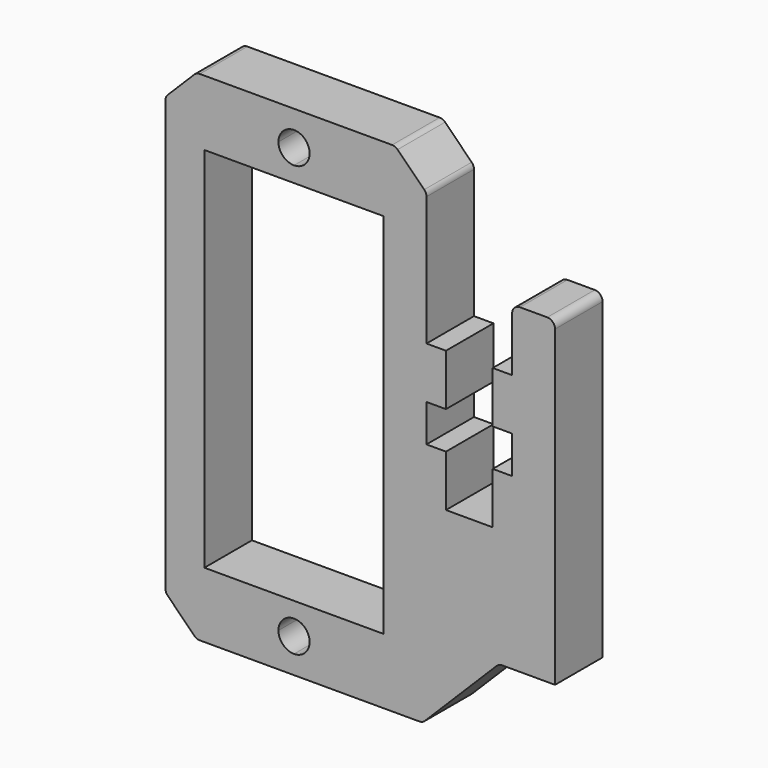
from build123d import *

# Parameters (mm, degrees)
F1_DEPTH = 3.81


# Not quite as in the source:
# - ends of sketch curves that miss each other by under 0.0002 mm in the source are joined


with BuildPart() as f1:
    # F0 (on Front) → F1 (new body)
    with BuildSketch(Plane.XZ):
        with BuildLine():
            Line((-10.292893, -16), (-4.25, -16))
            Line((-4.25, -16), (-4.25, -14.8))
            ThreePointArc((-4.25, -14.8), (-4.9571067812, -14.5071067812), (-5.25, -13.8))
            ThreePointArc((-5.25, -13.8), (-4.9571067812, -13.0928932188), (-4.25, -12.8))
            Line((-4.25, -12.8), (-4.25, -11.8))
            Line((-4.25, -11.8), (-10, -11.8))
            Line((-10, -11.8), (-10, 11.8))
            Line((-10, 11.8), (-4.25, 11.8))
            Line((-4.25, 11.8), (-4.25, 12.8))
            ThreePointArc((-4.25, 12.8), (-4.9571067812, 13.0928932188), (-5.25, 13.8))
            ThreePointArc((-5.25, 13.8), (-4.9571067812, 14.5071067812), (-4.25, 14.8))
            Line((-4.25, 14.8), (-4.25, 16))
            Line((-4.25, 16), (-10.292893, 16))
            ThreePointArc((-10.292893, 16), (-10.4842347162, 15.9619397663), (-10.6464463906, 15.8535533906))
            Line((-10.6464463906, 15.8535533906), (-12.353554, 14.146447))
            ThreePointArc((-12.353554, 14.146447), (-12.4619399016, 13.9842353895), (-12.5, 13.792894))
            Line((-12.5, 13.792894), (-12.5, -13.792893))
            ThreePointArc((-12.5, -13.792893), (-12.4619399016, -13.9842343895), (-12.3535538906, -14.1464458906))
            Line((-12.3535538906, -14.1464458906), (-10.646447, -15.853553))
            ThreePointArc((-10.646447, -15.853553), (-10.4842350428, -15.961939631), (-10.292893, -16))
        make_face()
        with BuildLine():
            Line((12.5, -11.1), (12.5, 9))
            ThreePointArc((12.5, 9), (12.3535533906, 9.3535533906), (12, 9.5))
            Line((12, 9.5), (10.25, 9.5))
            ThreePointArc((10.25, 9.5), (9.8964466094, 9.3535533906), (9.75, 9))
            Line((9.75, 9), (9.75, 5.5))
            Line((9.75, 5.5), (8.5, 5.5))
            Line((8.5, 5.5), (8.5, 2.2))
            Line((8.5, 2.2), (9.75, 2.2))
            Line((9.75, 2.2), (9.75, -0.2))
            Line((9.75, -0.2), (8.5, -0.2))
            Line((8.5, -0.2), (8.5, -3.5))
            Line((8.5, -3.5), (5.5, -3.5))
            Line((5.5, -3.5), (5.5, -0.2))
            Line((5.5, -0.2), (4.25, -0.2))
            Line((4.25, -0.2), (4.25, 2.2))
            Line((4.25, 2.2), (5.5, 2.2))
            Line((5.5, 2.2), (5.5, 5.5))
            Line((5.5, 5.5), (4.25, 5.5))
            Line((4.25, 5.5), (4.25, 13.792894))
            ThreePointArc((4.25, 13.792894), (4.2119397663, 13.9842357162), (4.1035533906, 14.1464473906))
            Line((4.1035533906, 14.1464473906), (2.396446, 15.853554))
            ThreePointArc((2.396446, 15.853554), (2.2342343895, 15.9619399016), (2.042893, 16))
            Line((2.042893, 16), (-4.25, 16))
            Line((-4.25, 16), (-4.25, 14.8))
            ThreePointArc((-4.25, 14.8), (-3.5428932188, 14.5071067812), (-3.25, 13.8))
            ThreePointArc((-3.25, 13.8), (-3.5428932188, 13.0928932188), (-4.25, 12.8))
            Line((-4.25, 12.8), (-4.25, 11.8))
            Line((-4.25, 11.8), (1.5, 11.8))
            Line((1.5, 11.8), (1.5, -11.8))
            Line((1.5, -11.8), (-4.25, -11.8))
            Line((-4.25, -11.8), (-4.25, -12.8))
            ThreePointArc((-4.25, -12.8), (-3.5428932188, -13.0928932188), (-3.25, -13.8))
            ThreePointArc((-3.25, -13.8), (-3.5428932188, -14.5071067812), (-4.25, -14.8))
            Line((-4.25, -14.8), (-4.25, -16))
            Line((-4.25, -16), (3.792893, -16))
            ThreePointArc((3.792893, -16), (3.9842347162, -15.9619397663), (4.1464463906, -15.8535533906))
            Line((4.1464463906, -15.8535533906), (8.753553, -11.246446))
            ThreePointArc((8.753553, -11.246446), (8.9157652838, -11.1380602337), (9.107107, -11.1))
            Line((9.107107, -11.1), (12.5, -11.1))
        make_face()
    extrude(amount=F1_DEPTH)


solid = f1.part
